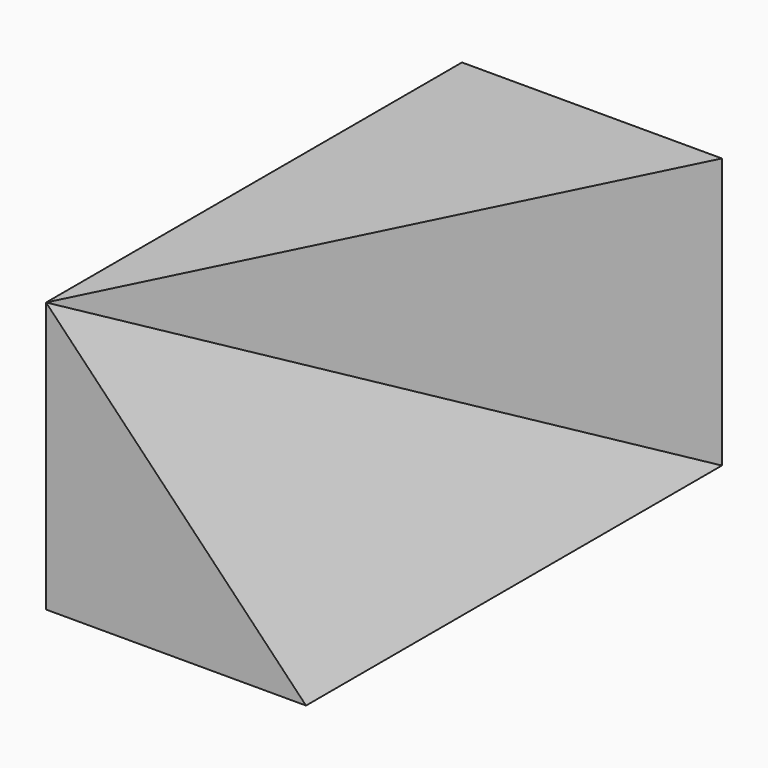
from build123d import *

# Parameters (mm, degrees)
F1_DEPTH = 52
F3_DEPTH = 100


# Not quite as in the source:
# - an extrude ends at something that could not be found from the text; its depth is read off the source's solid


with BuildPart() as f1:
    # F0 (on Top) → F1 (new body)
    with BuildSketch(Plane.XY):
        Polygon((0, 100), (0, 0), (50, 100), align=None)
    extrude(amount=F1_DEPTH)

    # F2 (on face) → F3 (join, through all)
    with BuildSketch(Plane(origin=(0, 100, 0), x_dir=(-1, 0, 0), z_dir=(0, 1, 0))):
        Polygon((0, 52), (-50, 0), (0, 0), align=None)
    extrude(amount=-F3_DEPTH)


solid = f1.part
